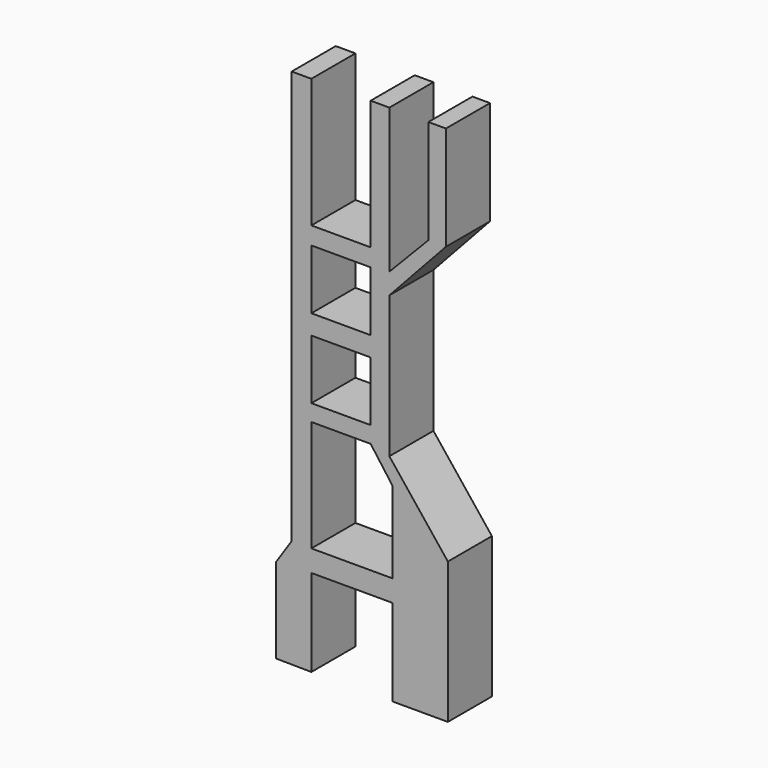
from build123d import *

# Parameters (mm, degrees)
F1_DEPTH = 10


# Not quite as in the source:
# - a feature of the source that left no trace in its solid (it failed there, or was rolled back) is left out


with BuildPart() as f1:
    # F0 (on Front) → F1 (new body)
    with BuildSketch(Plane.XZ):
        Polygon((-54.1052184999, 47.8023849428), (-57.6798580587, 47.8023849428), (-57.6798580587, -27.2650625557), (-60.5125948787, -31.5141640604), (-60.5125948787, -46.9525642693), (-54.1052184999, -47.0233857632), (-54.1052184999, -31.1857834458), (-39.3331050873, -31.1857834458), (-39.3331050873, -46.9423271716), (-29.3199270964, -46.9423271716), (-29.3199270964, -21.3033463806), (-39.9415493011, -7.9316543415), (-39.9415493011, 17.7926272154), (-29.6685695648, 28.9044026285), (-29.6685695648, 47.8023849428), (-32.8597128391, 47.8023849428), (-32.8597128391, 28.9044026285), (-39.9415493011, 21.5739104897), (-39.9415493011, 47.8023849428), (-43.3408282697, 47.8023849428), (-43.3408282697, 24.3615116924), (-54.1052184999, 24.3615116924), align=None)
        Polygon((-54.1052184999, -7.0560085587), (-43.3408282697, -7.0560085587), (-39.3331050873, -12.5158438459), (-39.3331050873, -27.2650625557), (-54.1052184999, -27.2650625557), align=None, mode=Mode.SUBTRACT)
        Polygon((-43.3408282697, 6.7588053644), (-43.3408282697, -1.2844107114), (-43.3408282697, -4.0514403954), (-54.1052184999, -4.0514403954), (-54.1052184999, 6.7588053644), align=None, mode=Mode.SUBTRACT)
        Polygon((-43.3408282697, 21.1618710309), (-43.3408282697, 11.6142081097), (-43.3408282697, 10.3236073628), (-54.1052184999, 10.3236073628), (-54.1052184999, 21.1618710309), align=None, mode=Mode.SUBTRACT)
    extrude(amount=F1_DEPTH)


solid = f1.part
